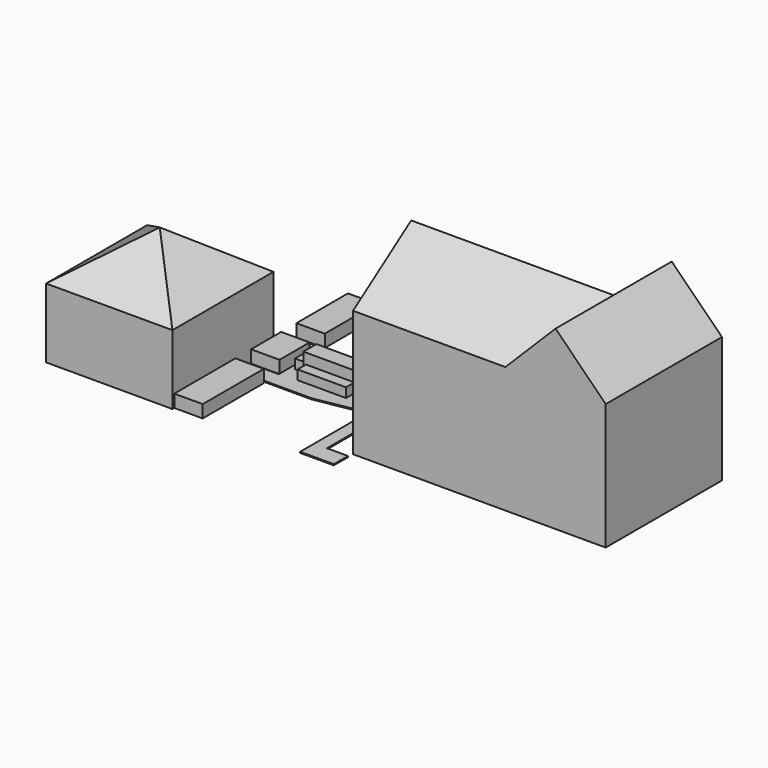
from build123d import *

# Parameters (mm, degrees)
F0_W      = 1371.6
F0_H      = 3684.9179491401
F1_DEPTH  = 609.6
F0_H_2    = 3113.3810096741
F2_DEPTH  = 5486.4
F3_SIZE2  = 2134.232566
F3_SIZE   = 3047.99999
F0_W_2    = 12192
F0_H_3    = 7010.4
F4_DEPTH  = 6096
F6_DEPTH  = 7010.4
F10_W     = 2336.8
F10_H     = 508
F11_DEPTH = 508
F10_W_2   = 508
F10_H_2   = 533.4
F10_W_3   = 603.8634702563
F10_H_3   = 1345.7531929016
F12_DEPTH = 1016
F14_DEPTH = 50.8


# Not quite as in the source:
# - a fillet or chamfer is up to 0.001 mm smaller than in the source, because OpenCascade refuses the exact size
# - the program builds the solid bodies; features that only make, move or delete a surface that nothing else refers to are left out


with BuildPart() as f1:
    # F0 (on Top) → F1 (new body)
    with BuildSketch(Plane.XY):
        with Locations((-6934.2, 1954.9984820187)):
            Rectangle(F0_W, F0_H)
    extrude(amount=F1_DEPTH)


with BuildPart() as f1b:
    # F0 (on Top) → F1, piece 2 (new body)
    with BuildSketch(Plane.XY):
        Polygon((-7620, 6561.6774559021), (-7620, 6096), (-7620, 4746.4752197266), (-6248.4, 4746.4752197266), (-6248.4, 6561.6774559021), align=None)
    extrude(amount=F1_DEPTH)


with BuildPart() as f1c:
    # F0 (on Top) → F1, piece 3 (new body)
    with BuildSketch(Plane.XY):
        with Locations((-6934.2, 9032.7679607391)):
            Rectangle(F0_W, F0_H_2)
    extrude(amount=F1_DEPTH)


with BuildPart() as f2:
    # F0 (on Top) → F2 (new body)
    with BuildSketch(Plane.XY):
        Polygon((-13716, 0), (-7620, 0), (-7620, 112.5395074487), (-7620, 3797.4574565887), (-7620, 4746.4752197266), (-7620, 6096), (-13716, 6096), align=None)
    extrude(amount=F2_DEPTH)

    # F3 (size 3048 and 2134.2325764632 in the source; OpenCascade refuses exactly that, so slightly less here)
    f3_edges = [f2.edges().sort_by_distance(p)[0] for p in [
        (-10668, 0, 5486.4),
        (-7620, 3048, 5486.4),
        (-10668, 6096, 5486.4),
        (-13716, 3048, 5486.4),
    ]]
    f3_side = f2.faces().sort_by_distance((-10668, 3048, 5486.4))[0]
    chamfer(f3_edges, length=F3_SIZE, length2=F3_SIZE2, reference=f3_side)


with BuildPart() as f4:
    # F0 (on Top) → F4 (new body)
    with BuildSketch(Plane.XY):
        with Locations((6096, 4876.8)):
            Rectangle(F0_W_2, F0_H_3)
    extrude(amount=F4_DEPTH)

    # F5 (on face) → F6 (join, through all)
    with BuildSketch(Plane.XZ.offset(-1371.6)):
        Polygon((7351.821556229, 6096), (12192, 6096), (9771.9107781145, 8516.0892218855), align=None)
    extrude(amount=-F6_DEPTH)

    # F7 (on face) → F8 (join, up to the next surface of F4)
    with BuildSketch(Plane(origin=(0, 0, 0), x_dir=(0, -1, 0), z_dir=(-1, 0, 0))):
        Polygon((-4876.8, 8509.5739364624), (-8382, 6096), (-1371.6, 6096), align=None)
    extrude(until=Until.NEXT, dir=(1, 0, 0))


with BuildPart() as f11:
    # F10 (on Top) → F11 (new body)
    with BuildSketch(Plane.XY):
        with Locations((-4179.8933044434, 6259.3952697754)):
            Rectangle(F10_W, F10_H)
    extrude(amount=F11_DEPTH)


with BuildPart() as f11b:
    # F10 (on Top) → F11, piece 2 (new body)
    with BuildSketch(Plane.XY):
        with Locations((-5729.2933044434, 5611.6952697754)):
            Rectangle(F10_W_2, F10_H_2)
    extrude(amount=F11_DEPTH)


with BuildPart() as f11c:
    # F10 (on Top) → F11, piece 3 (new body)
    with BuildSketch(Plane.XY):
        with Locations((-4179.8933044434, 4963.9952697754)):
            Rectangle(F10_W, F10_H)
    extrude(amount=F11_DEPTH)


with BuildPart() as f11d:
    # F10 (on Top) → F11, piece 4 (new body)
    with BuildSketch(Plane.XY):
        with Locations((-2630.4933044434, 5611.6952697754)):
            Rectangle(F10_W_2, F10_H_2)
    extrude(amount=F11_DEPTH)


with BuildPart() as f12:
    # F10 (on Top) → F12 (new body)
    with BuildSketch(Plane.XY):
        with Locations((-404.5735634863, 6098.7594127655)):
            Rectangle(F10_W_3, F10_H_3)
    extrude(amount=F12_DEPTH)


with BuildPart() as f12b:
    # F10 (on Top) → F12, piece 2 (new body)
    with BuildSketch(Plane.XY):
        Polygon((-5348.2933044434, 6005.3952697754), (-5475.2933044434, 6005.3952697754), (-5475.2933044434, 5878.3952697754), (-5475.2933044434, 5344.9952697754), (-5475.2933044434, 5217.9952697754), (-5348.2933044434, 5217.9952697754), (-3011.4933044434, 5217.9952697754), (-2884.4933044434, 5217.9952697754), (-2884.4933044434, 5344.9952697754), (-2884.4933044434, 5878.3952697754), (-2884.4933044434, 6005.3952697754), (-3011.4933044434, 6005.3952697754), align=None)
    extrude(amount=F12_DEPTH)


with BuildPart() as f14:
    # F13 (on Top) → F14 (new body)
    with BuildSketch(Plane.XY):
        Polygon((0, 4419.6), (0, 5334), (-830.4370045662, 5334), (-830.4370045662, 6693.6980781448), (-2003.8484761488, 6691.6584623371), (-3237.6575581537, 7344.5940092938), (-7525.3930091858, 7337.1410968098), (-7525.3930091858, 6612.8264071736), (-6208.9473012541, 6612.8264071736), (-6208.9473012541, 4649.5519282613), (-7525.3930091858, 4649.5519282613), (-7525.3930091858, 3889.7521495819), (-4019.5266004871, 3889.7521495819), (-1624.2101192474, 4312.1110725601), (-1624.2101192474, 3889.7521495819), (-1624.2101192474, 210.4274940615), (0, 210.4274940615), (0, 1068.1687307482), (-1014.6101192474, 1068.1687307482), (-1014.6101192474, 4419.6), align=None)
    extrude(amount=F14_DEPTH)


solid = Compound([f1.part, f1b.part, f1c.part, f2.part, f4.part, f11.part, f11b.part, f11c.part, f11d.part, f12.part, f12b.part, f14.part])
